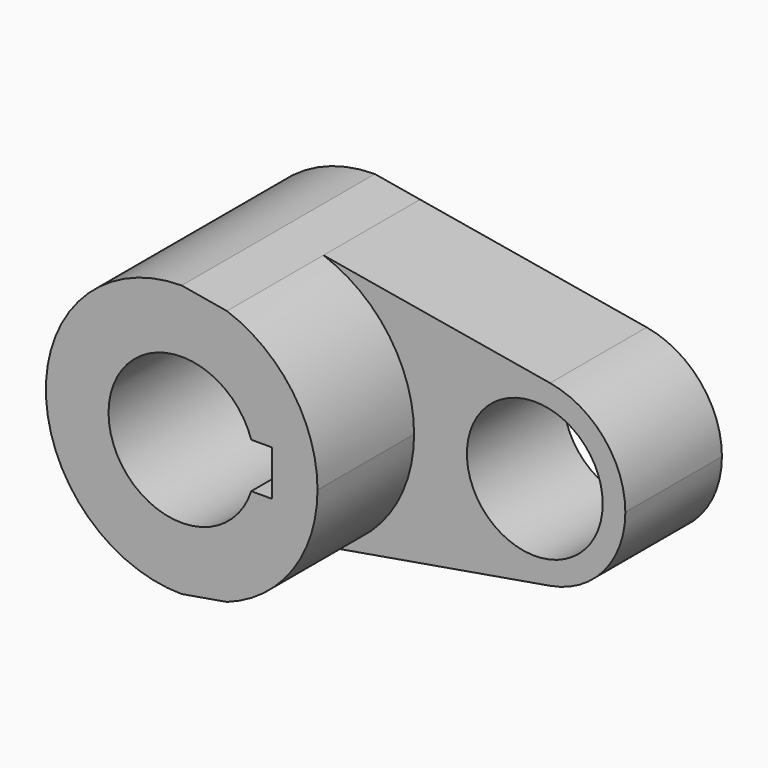
from build123d import *

# Parameters (mm, degrees)
F0_R     = 14.2875
F1_DEPTH = 25.4
F2_DEPTH = 50.8


with BuildPart() as f1:
    # F0 (on Front) → F1 (new body)
    with BuildSketch(Plane.XZ):
        with BuildLine():
            Line((9.5121844836, 26.9452959039), (0, 28.575))
            ThreePointArc((0, 28.575), (-28.575, 0), (0, -28.575))
            Line((0, -28.575), (9.5121844836, -26.9452959039))
            ThreePointArc((9.5121844836, -26.9452959039), (23.3274655355, -16.5033322905), (28.575, 0))
            ThreePointArc((28.575, 0), (23.3274655355, 16.5033322905), (9.5121844836, 26.9452959039))
        make_face()
        with BuildLine():
            ThreePointArc((-14.6329037383, 4.7625), (0, 15.3884137605), (14.6329037383, 4.7625))
            Line((14.6329037383, 4.7625), (19.05, 4.7625))
            Line((19.05, 4.7625), (19.05, -4.7625))
            Line((19.05, -4.7625), (14.6329037383, -4.7625))
            ThreePointArc((14.6329037383, -4.7625), (0, -15.3884137605), (-14.6329037383, -4.7625))
            Line((-14.6329037383, -4.7625), (-19.05, -4.7625))
            Line((-19.05, -4.7625), (-19.05, 4.7625))
            Line((-19.05, 4.7625), (-14.6329037383, 4.7625))
        make_face(mode=Mode.SUBTRACT)
        with BuildLine():
            Line((57.1919272622, 18.7764181619), (9.5121844836, 26.9452959039))
            ThreePointArc((9.5121844836, 26.9452959039), (23.3274655355, 16.5033322905), (28.575, 0))
            ThreePointArc((28.575, 0), (23.3274655355, -16.5033322905), (9.5121844836, -26.9452959039))
            Line((9.5121844836, -26.9452959039), (57.1919272622, -18.7764181619))
            ThreePointArc((57.1919272622, -18.7764181619), (34.925, 0), (57.1919272622, 18.7764181619))
        make_face()
        with BuildLine():
            ThreePointArc((73.025, 0), (68.5383952831, 12.2804730295), (57.1919272622, 18.7764181619))
            ThreePointArc((57.1919272622, 18.7764181619), (34.925, 0), (57.1919272622, -18.7764181619))
            ThreePointArc((57.1919272622, -18.7764181619), (68.5383952831, -12.2804730295), (73.025, 0))
        make_face()
        with Locations((53.975, 0)):
            Circle(F0_R, mode=Mode.SUBTRACT)
        with BuildLine():
            ThreePointArc((-14.6329037383, -4.7625), (-15.3884137605, 0), (-14.6329037383, 4.7625))
            Line((-14.6329037383, 4.7625), (-19.05, 4.7625))
            Line((-19.05, 4.7625), (-19.05, -4.7625))
            Line((-19.05, -4.7625), (-14.6329037383, -4.7625))
        make_face()
    extrude(amount=F1_DEPTH)

    # F0 (on Front) → F2 (join)
    with BuildSketch(Plane.XZ):
        with BuildLine():
            Line((9.5121844836, 26.9452959039), (0, 28.575))
            ThreePointArc((0, 28.575), (-28.575, 0), (0, -28.575))
            Line((0, -28.575), (9.5121844836, -26.9452959039))
            ThreePointArc((9.5121844836, -26.9452959039), (23.3274655355, -16.5033322905), (28.575, 0))
            ThreePointArc((28.575, 0), (23.3274655355, 16.5033322905), (9.5121844836, 26.9452959039))
        make_face()
        with BuildLine():
            ThreePointArc((-14.6329037383, 4.7625), (0, 15.3884137605), (14.6329037383, 4.7625))
            Line((14.6329037383, 4.7625), (19.05, 4.7625))
            Line((19.05, 4.7625), (19.05, -4.7625))
            Line((19.05, -4.7625), (14.6329037383, -4.7625))
            ThreePointArc((14.6329037383, -4.7625), (0, -15.3884137605), (-14.6329037383, -4.7625))
            Line((-14.6329037383, -4.7625), (-19.05, -4.7625))
            Line((-19.05, -4.7625), (-19.05, 4.7625))
            Line((-19.05, 4.7625), (-14.6329037383, 4.7625))
        make_face(mode=Mode.SUBTRACT)
        with BuildLine():
            ThreePointArc((-14.6329037383, -4.7625), (-15.3884137605, 0), (-14.6329037383, 4.7625))
            Line((-14.6329037383, 4.7625), (-19.05, 4.7625))
            Line((-19.05, 4.7625), (-19.05, -4.7625))
            Line((-19.05, -4.7625), (-14.6329037383, -4.7625))
        make_face()
    extrude(amount=F2_DEPTH)


solid = f1.part
